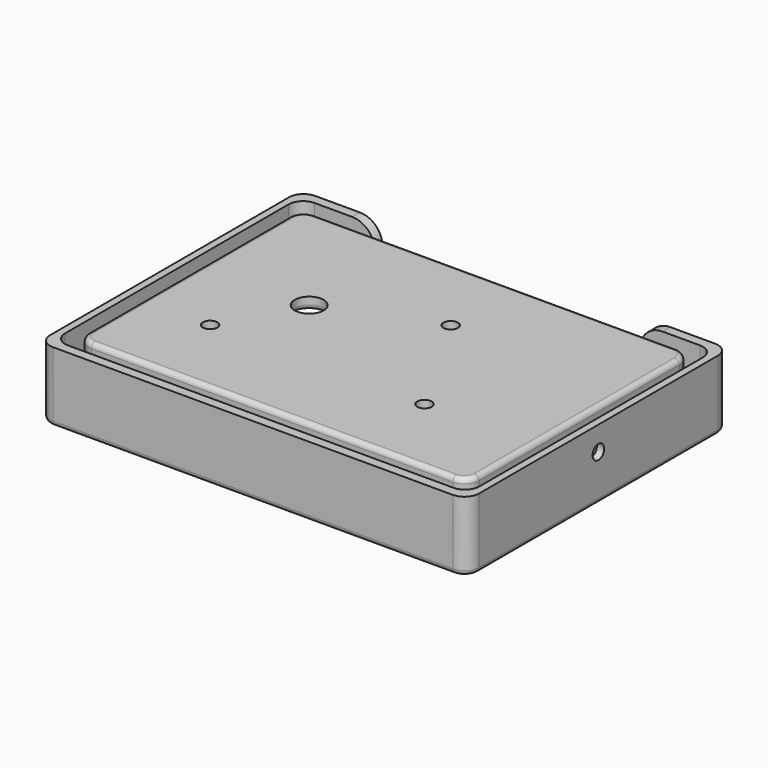
from build123d import *

# Parameters (mm, degrees)
F0_W          = 81
F0_H          = 58
F1_DEPTH      = 2.5
F2_R          = 1.5
F2_R_2        = 3
F3_DEPTH      = 25
F4_W          = 2
F4_H          = 2
F4_W_2        = 77
F4_H_2        = 54
F5_DEPTH      = 12
F6_W          = 89
F6_H          = 2
F7_DEPTH      = 5
F7_DEPTH_BACK = 63
F8_W          = 77
F8_H          = 54
F9_DEPTH      = 2
F10_W         = 1.5
F10_H         = 2
F10_W_2       = 86
F10_H_2       = 64
F11_DEPTH     = 12.5
F12_W         = 55
F12_H         = 14
F13_DEPTH     = 2
F14_R         = 4.7
F15_R         = 3
F16_R         = 1.5
F17_DEPTH     = 89.001
F18_R         = 3
F19_R         = 0.99999
F20_R         = 1


# Not quite as in the source:
# - a fillet or chamfer is up to 0.001 mm smaller than in the source, because OpenCascade refuses the exact size


with BuildPart() as f1:
    # F0 (on Top) → F1 (new body)
    with BuildSketch(Plane.XY):
        Rectangle(F0_W, F0_H)
    extrude(amount=F1_DEPTH)

    # F2 (on face) → F3 (cut)
    with BuildSketch(Plane.XY.offset(2.5)):
        with Locations((-26.5, -12)):
            Circle(F2_R)
        with Locations((18, -12)):
            Circle(F2_R)
        with Locations((4.0308988764, 12.2665245513)):
            Circle(F2_R)
        with Locations((-18.2936321066, 3.4565690241)):
            Circle(F2_R_2)
    extrude(amount=-F3_DEPTH, mode=Mode.SUBTRACT)

    # F4 (on face) → F5 (join)
    with BuildSketch(Plane(origin=(0, 0, 0), x_dir=(1, 0, 0), z_dir=(0, 0, -1))):
        with Locations((-39.5, 28)):
            Rectangle(F4_W, F4_H)
        with Locations((0, 28)):
            Rectangle(F4_W_2, F4_H)
        with Locations((-39.5, 0)):
            Rectangle(F4_W, F4_H_2)
        with Locations((39.5, 28)):
            Rectangle(F4_W, F4_H)
        with Locations((-39.5, -28)):
            Rectangle(F4_W, F4_H)
        with Locations((39.5, 0)):
            Rectangle(F4_W, F4_H_2)
        with Locations((0, -28)):
            Rectangle(F4_W_2, F4_H)
        with Locations((39.5, -28)):
            Rectangle(F4_W, F4_H)
    extrude(amount=F5_DEPTH)

    # F6 (on face) → F7 (join, two sides)
    with BuildSketch(Plane.XZ.offset(29)) as f7_sk:
        with Locations((0, -11)):
            Rectangle(F6_W, F6_H)
    extrude(amount=F7_DEPTH)
    extrude(f7_sk.sketch, amount=-F7_DEPTH_BACK)

    # F8 (on face) → F9 (cut, through all)
    with BuildSketch(Plane(origin=(0, 0, -12), x_dir=(1, 0, 0), z_dir=(0, 0, -1))):
        Rectangle(F8_W, F8_H)
    extrude(amount=-F9_DEPTH, mode=Mode.SUBTRACT)

    # F10 (on face) → F11 (join)
    with BuildSketch(Plane.XY.offset(-10)):
        with Locations((-43.75, -33)):
            Rectangle(F10_W, F10_H)
        with Locations((0, -33)):
            Rectangle(F10_W_2, F10_H)
        with Locations((-43.75, 0)):
            Rectangle(F10_W, F10_H_2)
        with Locations((43.75, -33)):
            Rectangle(F10_W, F10_H)
        with Locations((-43.75, 33)):
            Rectangle(F10_W, F10_H)
        with Locations((43.75, 0)):
            Rectangle(F10_W, F10_H_2)
        with Locations((0, 33)):
            Rectangle(F10_W_2, F10_H)
        with Locations((43.75, 33)):
            Rectangle(F10_W, F10_H)
    extrude(amount=F11_DEPTH)

    # F12 (on face) → F13 (cut)
    with BuildSketch(Plane(origin=(0, 34, 0), x_dir=(-1, 0, 0), z_dir=(0, 1, 0))):
        Rectangle(F12_W, F12_H)
    extrude(amount=-F13_DEPTH, mode=Mode.SUBTRACT)

    # F14
    f14_edges = [f1.edges().sort_by_distance(p)[0] for p in [
        (27.5, 33, -7),
        (-27.5, 33, -7),
        (27.5, 33, 2.5),
        (-27.5, 33, 2.5),
    ]]
    fillet(f14_edges, radius=F14_R)

    # F15
    f15_edges = [f1.edges().sort_by_distance(p)[0] for p in [
        (40.5, -29, -3.75),
        (-40.5, -29, -3.75),
        (40.5, 29, -3.75),
        (-40.5, 29, -3.75),
        (38.5, 27, -6),
        (-38.5, 27, -6),
        (-38.5, -27, -6),
        (38.5, -27, -6),
        (44.5, 34, -4.75),
        (-44.5, -34, -4.75),
        (44.5, -34, -4.75),
        (-44.5, 34, -4.75),
    ]]
    fillet(f15_edges, radius=F15_R)

    # F16 (on face) → F17 (cut, through all)
    with BuildSketch(Plane(origin=(-44.5, 0, 0), x_dir=(0, -1, 0), z_dir=(-1, 0, 0))):
        with Locations((0, -2.5)):
            Circle(F16_R)
    extrude(amount=-F17_DEPTH, mode=Mode.SUBTRACT)

    # F18
    f18_edges = [f1.edges().sort_by_distance(p)[0] for p in [
        (43, -32, -3.75),
        (-43, -32, -3.75),
        (43, 32, -3.75),
        (-43, 32, -3.75),
    ]]
    fillet(f18_edges, radius=F18_R)

    # F19 (radius 1 in the source; OpenCascade refuses exactly that, so slightly less here)
    f19_edges = [f1.edges().sort_by_distance(p)[0] for p in [
        (0, -29, 2.5),
        (0, 27, 0),
        (0, 27, -12),
        (0, 34, -12),
    ]]
    fillet(f19_edges, radius=F19_R)

    # F20
    f20_edges = [f1.edges().sort_by_distance(p)[0] for p in [
        (-21.293632, 3.456569, 0),
    ]]
    fillet(f20_edges, radius=F20_R)


solid = f1.part
